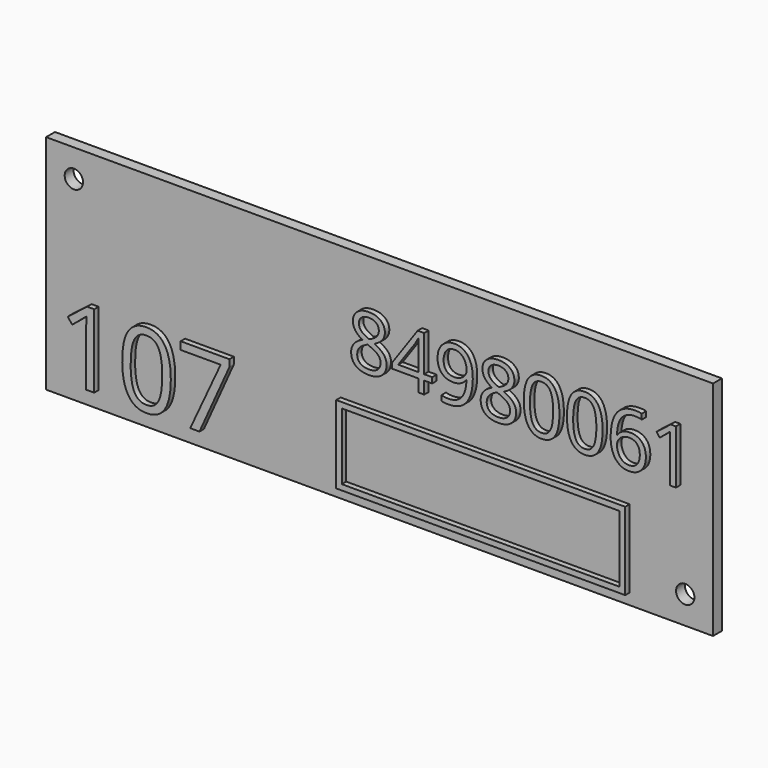
from build123d import *

# Parameters (mm, degrees)
F0_W         = 120
F0_H         = 40
F1_DEPTH     = 2
F3_D         = 3.3
F4_TEXT_SIZE = 13.5871488217
F5_DEPTH     = 1
F6_TEXT_SIZE = 18.5054667028
F7_DEPTH     = 1
F8_W         = 52
F8_H         = 14
F8_W_2       = 49.99999962
F8_H_2       = 11.99999962
F9_DEPTH     = 1


# Not quite as in the source:
# - Text() gives the source's letters only with a copy of the font that has no kerning and outlines rounded to 1/6400 em; it was checked with that copy


with BuildPart() as f1:
    # F0 (on Front) → F1 (new body)
    with BuildSketch(Plane.XZ):
        Rectangle(F0_W, F0_H)
    extrude(amount=F1_DEPTH)

    # F3 (through all)
    with Locations(Plane.XZ.offset(2)):
        with Locations((-55, 15), (55, -15)):
            Hole(F3_D / 2)

    # F4 (on face) → F5 (join)
    with BuildSketch(Plane.XZ.offset(2)):
        with Locations((-5, 2)):
            Text('84980061', F4_TEXT_SIZE, font='Open Sans', text_align=(TextAlign.LEFT, TextAlign.BOTTOM))
    extrude(amount=F5_DEPTH)

    # F6 (on face) → F7 (join)
    with BuildSketch(Plane.XZ.offset(2)):
        with Locations((-57, -17)):
            Text('107', F6_TEXT_SIZE, font='Open Sans', text_align=(TextAlign.LEFT, TextAlign.BOTTOM))
    extrude(amount=F7_DEPTH)

    # F8 (on face) → F9 (join)
    with BuildSketch(Plane.XZ.offset(2)):
        with Locations((19, -11)):
            Rectangle(F8_W, F8_H)
        with Locations((19, -11)):
            Rectangle(F8_W_2, F8_H_2, mode=Mode.SUBTRACT)
    extrude(amount=F9_DEPTH)


solid = f1.part
